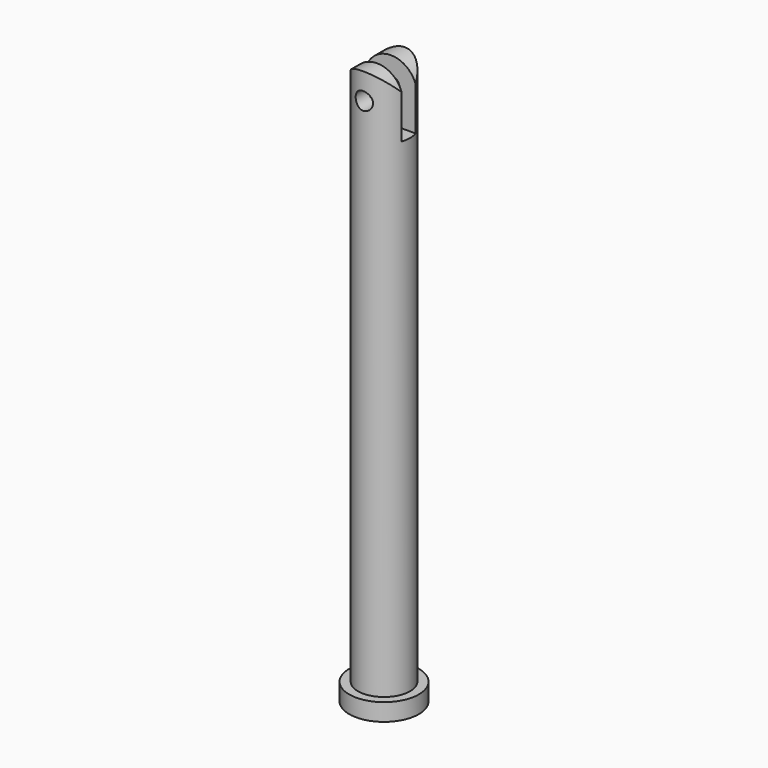
from build123d import *

# Parameters (mm, degrees)
F0_R          = 4.7625
F1_DEPTH      = 101.6
F2_W          = 9.525
F2_H          = 3.175
F3_DEPTH      = 12.7
F4_R          = 1.5875
F5_DEPTH      = 151
F5_DEPTH_BACK = 151
F6_R          = 6.35
F7_DEPTH      = 3.175


# Not quite as in the source:
# - an extrude ends at something that could not be found from the text; its depth is read off the source's solid


with BuildPart() as f1:
    # F0 (on Top) → F1 (new body)
    with BuildSketch(Plane.XY):
        Circle(F0_R)
    extrude(amount=F1_DEPTH)

    # F2 (on face) → F3 (cut)
    with BuildSketch(Plane.XY.offset(101.6)):
        Rectangle(F2_W, F2_H)
    extrude(amount=-F3_DEPTH, mode=Mode.SUBTRACT)

    # F4 (on Front) → F5 (cut, two sides)
    with BuildSketch(Plane.XZ) as f5_sk:
        with BuildLine():
            Line((4.7625, 101.6), (-4.7625, 101.6))
            Line((-4.7625, 101.6), (-4.7625, 95.25))
            ThreePointArc((-4.7625, 95.25), (0, 100.0125), (4.7625, 95.25))
            Line((4.7625, 95.25), (4.7625, 101.6))
        make_face()
        with Locations((0, 95.25)):
            Circle(F4_R)
    extrude(amount=-F5_DEPTH, mode=Mode.SUBTRACT)
    extrude(f5_sk.sketch, amount=F5_DEPTH_BACK, mode=Mode.SUBTRACT)

    # F6 (on face) → F7 (join)
    with BuildSketch(Plane(origin=(0, 0, 0), x_dir=(1, 0, 0), z_dir=(0, 0, -1))):
        Circle(F6_R)
    extrude(amount=F7_DEPTH)


solid = f1.part
